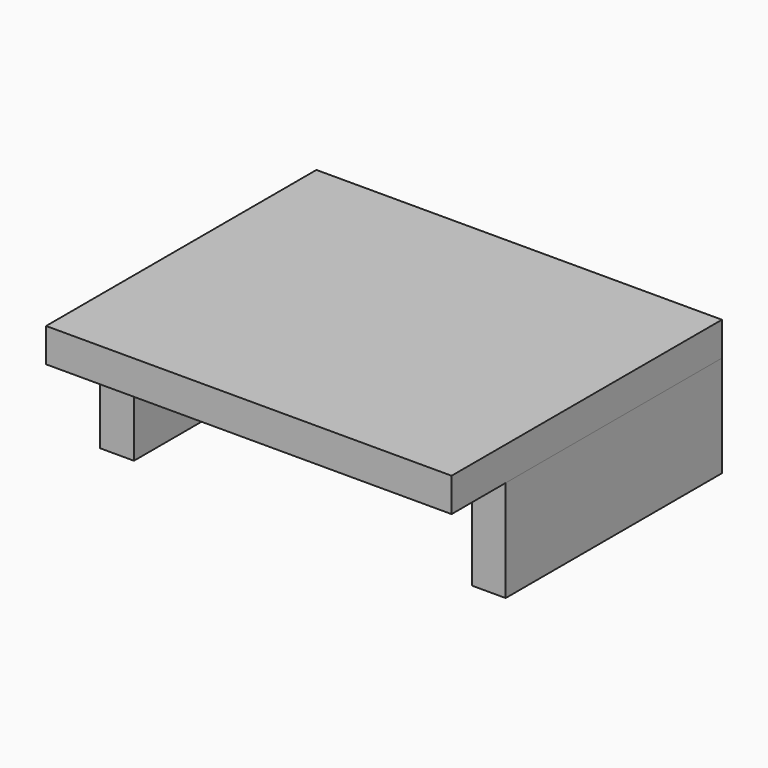
from build123d import *

# Parameters (mm, degrees)
F0_W     = 3.175
F0_H     = 3.175
F0_W_2   = 31.7499573946
F0_W_3   = 3.1750426054
F1_DEPTH = 31.75
F0_H_2   = 9.525
F2_DEPTH = 25.4


# Not quite as in the source:
# - ends of sketch curves that miss each other by under 0.0002 mm in the source are joined


with BuildPart() as f1:
    # F0 (on Front) → F1 (new body)
    with BuildSketch(Plane.XZ):
        with Locations((-17.4625, 23.0930101633)):
            Rectangle(F0_W, F0_H)
        with Locations((-2.13027e-05, 23.0930101633)):
            Rectangle(F0_W_2, F0_H)
        with Locations((17.4624786973, 23.0930101633)):
            Rectangle(F0_W_3, F0_H)
    extrude(amount=F1_DEPTH)


with BuildPart() as f2:
    # F0 (on Front) → F2 (new body)
    with BuildSketch(Plane.XZ):
        with Locations((-17.4625, 16.7430101633)):
            Rectangle(F0_W, F0_H_2)
    extrude(amount=F2_DEPTH)


with BuildPart() as f2b:
    # F0 (on Front) → F2, piece 2 (new body)
    with BuildSketch(Plane.XZ):
        Polygon((19.05, 21.5055101633), (15.8749573946, 21.5055101633), (15.8749573946, 11.9805101633), (19.0499573946, 11.9805101633), align=None)
    extrude(amount=F2_DEPTH)


solid = Compound([f1.part, f2.part, f2b.part])
